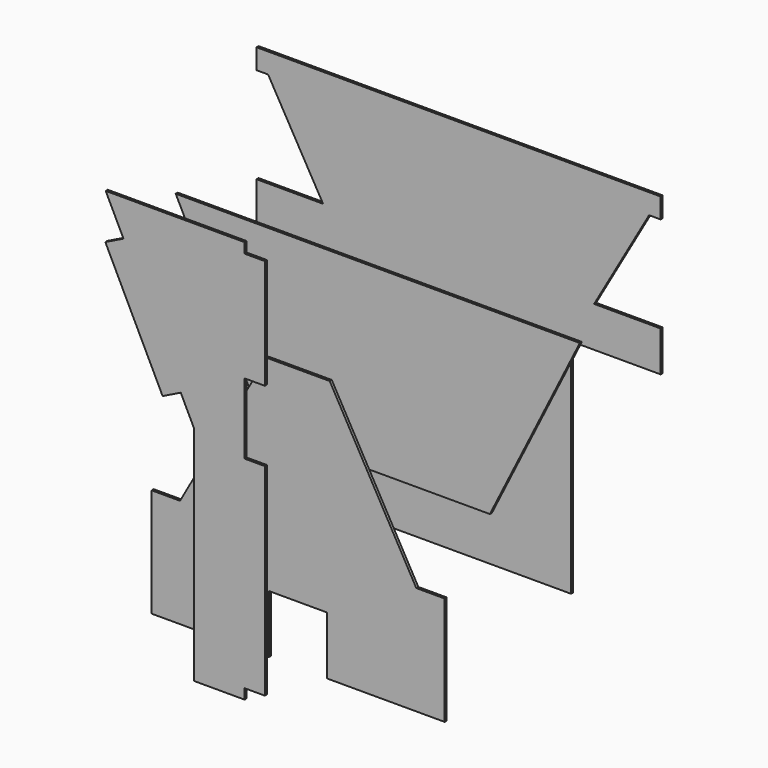
from build123d import *

# Parameters (mm, degrees)
F1_DEPTH  = 3.175
F3_W      = 25.4
F3_H      = 254
F3_H_2    = 137.9474
F4_DEPTH  = 3.175
F7_DEPTH  = 3.175
F9_W      = 282.575
F9_H      = 279.4
F10_DEPTH = 3.175


# Not quite as in the source:
# - a length typed as a fraction of an inch, garbled in the dataset ("3 / 203.2 mm" for 3/8 in), is restored


with BuildPart() as f1:
    # F0 (on Front) → F1 (new body)
    with BuildSketch(Plane.XZ):
        Polygon((36.5125, 165.1), (-36.5125, 165.1), (-39.6875, 165.1), (-148.4802469136, -28.575), (-184.15, -28.575), (-184.15, -92.075), (-184.15, -165.1), (-36.5125, -165.1), (-36.5125, -92.075), (36.5125, -92.075), (36.5125, -165.1), (184.15, -165.1), (184.15, -92.075), (184.15, -28.575), (148.4802469136, -28.575), (39.6875, 165.1), align=None)
    extrude(amount=F1_DEPTH)


with BuildPart() as f4:
    # F3 (on offset) → F4 (new body)
    with BuildSketch(Plane(origin=(0, -127, 0), x_dir=(-1, 0, 0), z_dir=(0, 1, 0))):
        Polygon((31.75, -139.7), (31.75, 139.7), (-31.75, 139.7), (-31.75, 127), (-31.75, -127), (-31.75, -139.7), align=None)
        Polygon((-31.75, 139.7), (31.75, 139.7), (48.5109045543, 173.9152316742), (120.5271272609, 320.927091101), (142.875, 366.5474), (-31.75, 366.5474), (-31.75, 353.8474), (-31.75, 215.9), align=None)
        Polygon((120.5271272609, 320.927091101), (48.5109045543, 173.9152316742), (71.3210590038, 162.7412953047), (143.3372817104, 309.7531547315), align=None)
        with Locations((-44.45, 0)):
            Rectangle(F3_W, F3_H)
        with Locations((-44.45, 284.8737)):
            Rectangle(F3_W, F3_H_2)
    extrude(amount=F4_DEPTH)


with BuildPart() as f7:
    # F6 (on offset) → F7 (new body)
    with BuildSketch(Plane(origin=(0, 121.92, 0), x_dir=(-1, 0, 0), z_dir=(0, 1, 0))):
        Polygon((254, 226.0501956), (0, 226.0501956), (-254, 226.0501956), (-140.9192, 0), (0, 0), (140.9192, 0), align=None)
    extrude(amount=F7_DEPTH)


with BuildPart() as f10:
    # F9 (on offset) → F10 (new body)
    with BuildSketch(Plane(origin=(0, 248.92, 0), x_dir=(-1, 0, 0), z_dir=(0, 1, 0))):
        Rectangle(F9_W, F9_H)
        Polygon((-0.0127, 15.875), (-63.5127, 15.875), (-63.5127, 101.6), (-0.0127, 101.6), (63.4873, 101.6), (63.4873, 15.875), align=None, mode=Mode.SUBTRACT)
        Polygon((-170.3745967742, 190.5), (-141.2875, 139.7), (141.2875, 139.7), (170.3745967742, 190.5), (239.4564516129, 311.15), (254, 336.55), (-254, 336.55), (-239.4564516129, 311.15), align=None)
        Polygon((-254, 139.7), (-141.2875, 139.7), (-170.3745967742, 190.5), (-254, 190.5), align=None)
        Polygon((170.3745967742, 190.5), (141.2875, 139.7), (254, 139.7), (254, 190.5), align=None)
        Polygon((254, 336.55), (239.4564516129, 311.15), (254, 311.15), align=None)
        Polygon((-254, 311.15), (-239.4564516129, 311.15), (-254, 336.55), align=None)
    extrude(amount=F10_DEPTH)


solid = Compound([f1.part, f4.part, f7.part, f10.part])
